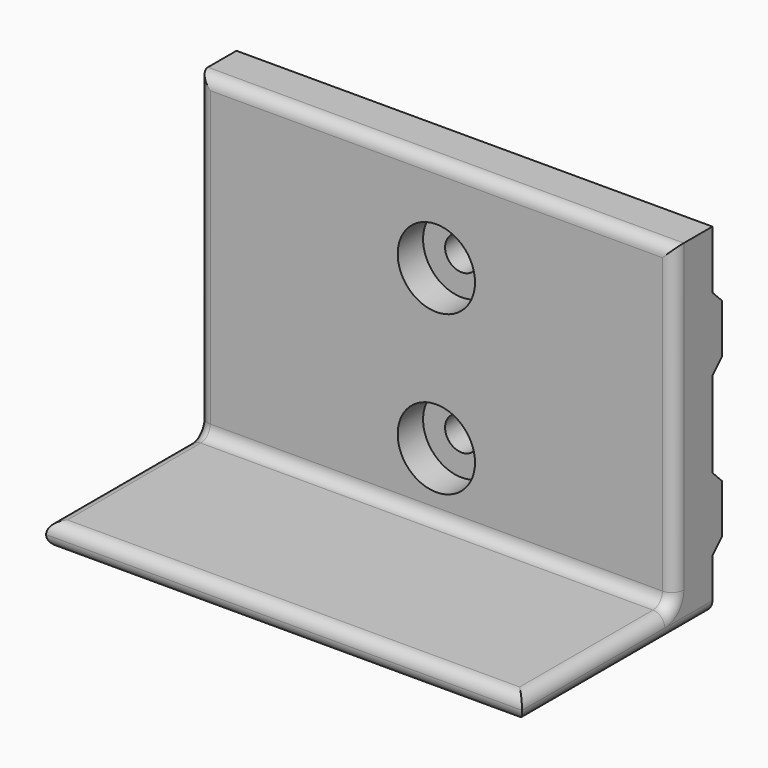
from build123d import *

# Parameters (mm, degrees)
F1_DEPTH       = 60
F2_R           = 1.49999
F4_D           = 4.2
F4_CBORE_D     = 9.75
F4_CBORE_DEPTH = 4


# Not quite as in the source:
# - a fillet or chamfer is up to 0.001 mm smaller than in the source, because OpenCascade refuses the exact size
# - a feature names something its author has since deleted; it is built from what else it names


with BuildPart() as f1:
    # F0 (on Right) → F1 (new body)
    with BuildSketch(Plane.YZ):
        Polygon((10, 1.9290046394), (4, 1.9290046394), (4, -38.0709953606), (-20, -38.0709953606), (-20, -41.0709953606), (10, -41.0709953606), (10, -34.6), (11.5, -33.1), (11.5, -26.9), (10, -25.4), (10, -14.6), (11.5, -13.1), (11.5, -6.9), (10, -5.4), align=None)
    extrude(amount=-F1_DEPTH)

    # F2 (radius 1.5 in the source; OpenCascade refuses exactly that, so slightly less here)
    f2_edges = [f1.edges().sort_by_distance(p)[0] for p in [
        (0, 4, -18.070995),
        (-60, 4, -18.070995),
        (0, -8, -38.070995),
        (-30, -20, -38.070995),
        (-60, -8, -38.070995),
        (-30, 4, -38.070995),
        (-30, -20, -41.070995),
        (0, -5, -41.070995),
        (-60, -5, -41.070995),
        (-30, 4, 1.929005),
    ]]
    fillet(f2_edges, radius=F2_R)

    # F4 (through all)
    with Locations(Plane.XZ.offset(-4)):
        with Locations((-30, -9.9999953606), (-30, -29.9999953606)):
            CounterBoreHole(F4_D / 2, F4_CBORE_D / 2, F4_CBORE_DEPTH)


solid = f1.part
